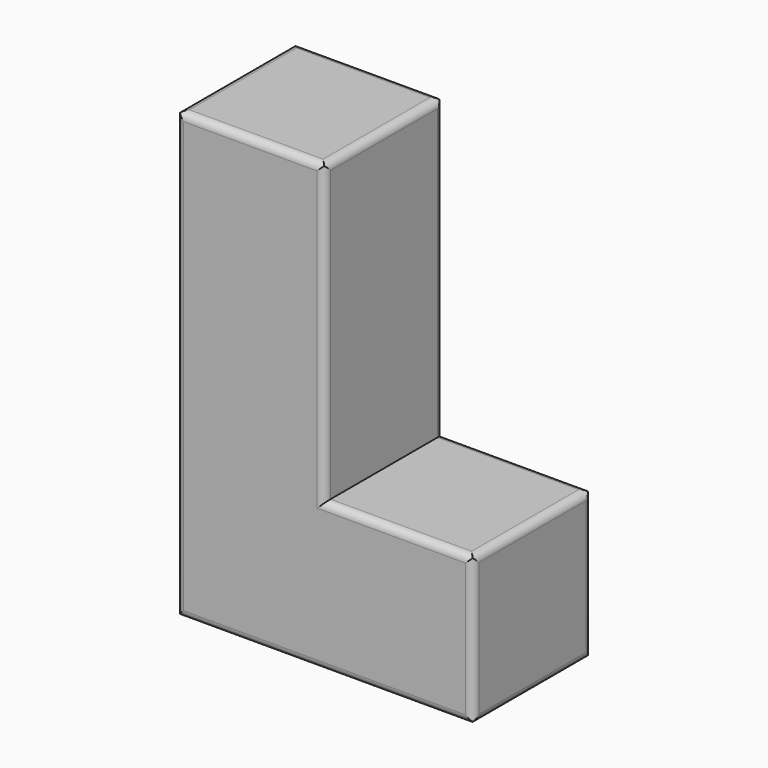
from build123d import *

# Parameters (mm, degrees)
F0_W        = 10
F0_H        = 10
F1_DEPTH    = 10
F2_R        = 0.5
F3_T1_DEPTH = 11.5


# Not quite as in the source:
# - a fillet or chamfer that OpenCascade refuses, or shapes differently, is made with other operations: its cross-section is extruded or revolved along the edge and cut away or added


with BuildPart() as f1:
    # F0 (on Front) → F1 (new body)
    with BuildSketch(Plane.XZ):
        Polygon((5, 15), (-5, 15), (-5, -15), (5, -15), (5, -5), align=None)
        with Locations((10, -10)):
            Rectangle(F0_W, F0_H)
    extrude(amount=F1_DEPTH)

    # F2
    f2_edges = [f1.edges().sort_by_distance(p)[0] for p in [
        (0, -10, 15),
        (-5, -10, 0),
        (5, -10, -15),
        (15, -10, -10),
        (10, -10, -5),
        (5, -10, 5),
        (0, 0, 15),
        (-5, 0, 0),
        (5, 0, -15),
        (15, 0, -10),
        (10, 0, -5),
        (5, 0, 5),
    ]]
    fillet(f2_edges, radius=F2_R)

    # F3: fillet of radius 0.5 on 11 edges, made by hand

    # F3_s2 → F3_t1 (cut)
    with BuildSketch(Plane.XZ.offset(-0.75)):
        with BuildLine():
            ThreePointArc((-5, -14.5), (-4.8535533906, -14.8535533906), (-4.5, -15))
            Line((-4.5, -15), (-5, -15))
            Line((-5, -15), (-5, -14.5))
        make_face()
        with BuildLine():
            ThreePointArc((14.5, -15), (14.8535533906, -14.8535533906), (15, -14.5))
            Line((15, -14.5), (15, -15))
            Line((15, -15), (14.5, -15))
        make_face()
        with BuildLine():
            ThreePointArc((4.5, 15), (4.8535533906, 14.8535533906), (5, 14.5))
            Line((5, 14.5), (5, 15))
            Line((5, 15), (4.5, 15))
        make_face()
        with BuildLine():
            ThreePointArc((-4.5, 15), (-4.8535533906, 14.8535533906), (-5, 14.5))
            Line((-5, 14.5), (-5, 15))
            Line((-5, 15), (-4.5, 15))
        make_face()
        with BuildLine():
            ThreePointArc((14.5, -5), (14.8535533906, -5.1464466094), (15, -5.5))
            Line((15, -5.5), (15, -5))
            Line((15, -5), (14.5, -5))
        make_face()
    extrude(amount=F3_T1_DEPTH, mode=Mode.SUBTRACT)


solid = f1.part
